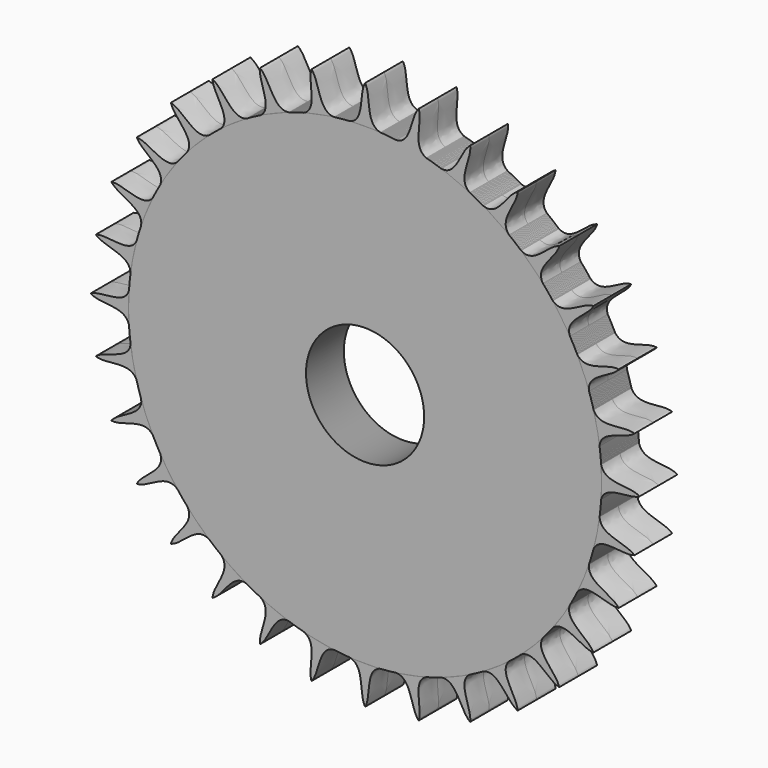
from build123d import *

# Parameters (mm, degrees)
F0_R     = 6.35
F1_DEPTH = 2.54
F2_COUNT = 32


with BuildPart() as f1:
    # F0 (on Front) → F1 (new body, symmetric)
    with BuildSketch(Plane.XZ):
        with BuildLine():
            add(Edge.make_bspline(
                [(-1.6565648674, 25.3459226078), (0, 25.7344954968), (-0.6848442595, 28.3242439591), (0, 29.4843787699)],
                knots=[0, 0, 0, 0, 4.4576929645, 4.4576929645, 4.4576929645, 4.4576929645], degree=3))
            ThreePointArc((-1.6565648674, 25.3459226078), (0, 25.4650093878), (1.6565648674, 25.3459226078))
            add(Edge.make_bspline(
                [(1.6565648674, 25.3459226078), (0, 25.7344954968), (0.6848442595, 28.3242439591), (0, 29.4843787699)],
                knots=[0, 0, 0, 0, 4.4576929645, 4.4576929645, 4.4576929645, 4.4576929645], degree=3))
        make_face()
        with BuildLine():
            ThreePointArc((1.6565648674, 25.3459226078), (0, 25.4650093878), (-1.6565648674, 25.3459226078))
            ThreePointArc((-1.6565648674, 25.3459226078), (0, 25.4), (1.6565648674, 25.3459226078))
        make_face()
        with BuildLine():
            ThreePointArc((1.6565648674, 25.3459226078), (0, 25.4), (-1.6565648674, 25.3459226078))
            ThreePointArc((-1.6565648674, 25.3459226078), (-17.3649539644, -18.5369461837), (25.4, 0))
            ThreePointArc((25.4, 0), (18.5369461837, 17.3649539644), (1.6565648674, 25.3459226078))
        make_face()
        Circle(F0_R, mode=Mode.SUBTRACT)
    extrude(amount=F1_DEPTH, both=True)


with BuildPart() as f2_1:
    # F2: instance of F1
    add(f1.part.rotate(Axis((0, 0, 0), (0, -1, 0)), 1 * 360 / F2_COUNT))


with BuildPart() as f2_2:
    # F2: instance of F1
    add(f1.part.rotate(Axis((0, 0, 0), (0, -1, 0)), 2 * 360 / F2_COUNT))


with BuildPart() as f2_3:
    # F2: instance of F1
    add(f1.part.rotate(Axis((0, 0, 0), (0, -1, 0)), 3 * 360 / F2_COUNT))


with BuildPart() as f2_4:
    # F2: instance of F1
    add(f1.part.rotate(Axis((0, 0, 0), (0, -1, 0)), 4 * 360 / F2_COUNT))


with BuildPart() as f2_5:
    # F2: instance of F1
    add(f1.part.rotate(Axis((0, 0, 0), (0, -1, 0)), 5 * 360 / F2_COUNT))


with BuildPart() as f2_6:
    # F2: instance of F1
    add(f1.part.rotate(Axis((0, 0, 0), (0, -1, 0)), 6 * 360 / F2_COUNT))


with BuildPart() as f2_7:
    # F2: instance of F1
    add(f1.part.rotate(Axis((0, 0, 0), (0, -1, 0)), 7 * 360 / F2_COUNT))


with BuildPart() as f2_8:
    # F2: instance of F1
    add(f1.part.rotate(Axis((0, 0, 0), (0, -1, 0)), 8 * 360 / F2_COUNT))


with BuildPart() as f2_9:
    # F2: instance of F1
    add(f1.part.rotate(Axis((0, 0, 0), (0, -1, 0)), 9 * 360 / F2_COUNT))


with BuildPart() as f2_10:
    # F2: instance of F1
    add(f1.part.rotate(Axis((0, 0, 0), (0, -1, 0)), 10 * 360 / F2_COUNT))


with BuildPart() as f2_11:
    # F2: instance of F1
    add(f1.part.rotate(Axis((0, 0, 0), (0, -1, 0)), 11 * 360 / F2_COUNT))


with BuildPart() as f2_12:
    # F2: instance of F1
    add(f1.part.rotate(Axis((0, 0, 0), (0, -1, 0)), 12 * 360 / F2_COUNT))


with BuildPart() as f2_13:
    # F2: instance of F1
    add(f1.part.rotate(Axis((0, 0, 0), (0, -1, 0)), 13 * 360 / F2_COUNT))


with BuildPart() as f2_14:
    # F2: instance of F1
    add(f1.part.rotate(Axis((0, 0, 0), (0, -1, 0)), 14 * 360 / F2_COUNT))


with BuildPart() as f2_15:
    # F2: instance of F1
    add(f1.part.rotate(Axis((0, 0, 0), (0, -1, 0)), 15 * 360 / F2_COUNT))


with BuildPart() as f2_16:
    # F2: instance of F1
    add(f1.part.rotate(Axis((0, 0, 0), (0, -1, 0)), 16 * 360 / F2_COUNT))


with BuildPart() as f2_17:
    # F2: instance of F1
    add(f1.part.rotate(Axis((0, 0, 0), (0, -1, 0)), 17 * 360 / F2_COUNT))


with BuildPart() as f2_18:
    # F2: instance of F1
    add(f1.part.rotate(Axis((0, 0, 0), (0, -1, 0)), 18 * 360 / F2_COUNT))


with BuildPart() as f2_19:
    # F2: instance of F1
    add(f1.part.rotate(Axis((0, 0, 0), (0, -1, 0)), 19 * 360 / F2_COUNT))


with BuildPart() as f2_20:
    # F2: instance of F1
    add(f1.part.rotate(Axis((0, 0, 0), (0, -1, 0)), 20 * 360 / F2_COUNT))


with BuildPart() as f2_21:
    # F2: instance of F1
    add(f1.part.rotate(Axis((0, 0, 0), (0, -1, 0)), 21 * 360 / F2_COUNT))


with BuildPart() as f2_22:
    # F2: instance of F1
    add(f1.part.rotate(Axis((0, 0, 0), (0, -1, 0)), 22 * 360 / F2_COUNT))


with BuildPart() as f2_23:
    # F2: instance of F1
    add(f1.part.rotate(Axis((0, 0, 0), (0, -1, 0)), 23 * 360 / F2_COUNT))


with BuildPart() as f2_24:
    # F2: instance of F1
    add(f1.part.rotate(Axis((0, 0, 0), (0, -1, 0)), 24 * 360 / F2_COUNT))


with BuildPart() as f2_25:
    # F2: instance of F1
    add(f1.part.rotate(Axis((0, 0, 0), (0, -1, 0)), 25 * 360 / F2_COUNT))


with BuildPart() as f2_26:
    # F2: instance of F1
    add(f1.part.rotate(Axis((0, 0, 0), (0, -1, 0)), 26 * 360 / F2_COUNT))


with BuildPart() as f2_27:
    # F2: instance of F1
    add(f1.part.rotate(Axis((0, 0, 0), (0, -1, 0)), 27 * 360 / F2_COUNT))


with BuildPart() as f2_28:
    # F2: instance of F1
    add(f1.part.rotate(Axis((0, 0, 0), (0, -1, 0)), 28 * 360 / F2_COUNT))


with BuildPart() as f2_29:
    # F2: instance of F1
    add(f1.part.rotate(Axis((0, 0, 0), (0, -1, 0)), 29 * 360 / F2_COUNT))


with BuildPart() as f2_30:
    # F2: instance of F1
    add(f1.part.rotate(Axis((0, 0, 0), (0, -1, 0)), 30 * 360 / F2_COUNT))


with BuildPart() as f2_31:
    # F2: instance of F1
    add(f1.part.rotate(Axis((0, 0, 0), (0, -1, 0)), 31 * 360 / F2_COUNT))


solid = Compound([f1.part, f2_1.part, f2_2.part, f2_3.part, f2_4.part, f2_5.part, f2_6.part, f2_7.part, f2_8.part, f2_9.part, f2_10.part, f2_11.part, f2_12.part, f2_13.part, f2_14.part, f2_15.part, f2_16.part, f2_17.part, f2_18.part, f2_19.part, f2_20.part, f2_21.part, f2_22.part, f2_23.part, f2_24.part, f2_25.part, f2_26.part, f2_27.part, f2_28.part, f2_29.part, f2_30.part, f2_31.part])
